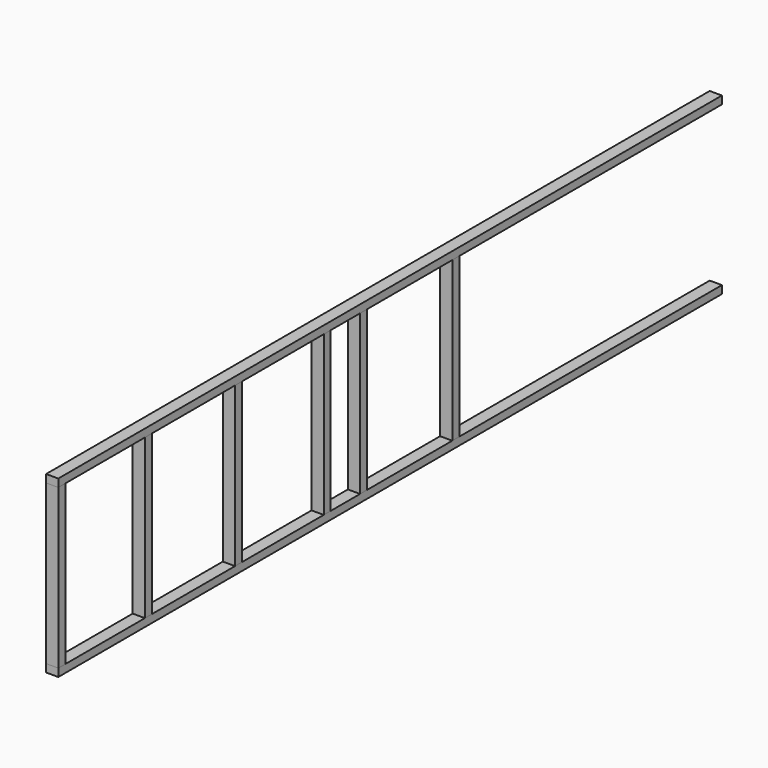
from build123d import *

# Parameters (mm, degrees)
F2_W     = 70
F2_H     = 45
F3_DEPTH = 2375
F4_W     = 50
F4_H     = 910.78125
F5_DEPTH = 70


with BuildPart() as f3:
    # F2 (on Front) → F3 (new body, symmetric)
    with BuildSketch(Plane.XZ):
        with Locations((-1245, 22.5)):
            Rectangle(F2_W, F2_H)
    extrude(amount=F3_DEPTH, both=True)


with BuildPart() as f3b:
    # F2 (on Front) → F3, piece 2 (new body, symmetric)
    with BuildSketch(Plane.XZ):
        with Locations((-1245, 978.28125)):
            Rectangle(F2_W, F2_H)
    extrude(amount=F3_DEPTH, both=True)


with BuildPart() as f5:
    # F4 (on face) → F5 (new body, through all)
    with BuildSketch(Plane(origin=(-1280, 0, 0), x_dir=(0, -1, 0), z_dir=(-1, 0, 0))):
        with Locations((2350, 500.390625)):
            Rectangle(F4_W, F4_H)
    extrude(amount=-F5_DEPTH)


with BuildPart() as f5b:
    # F4 (on face) → F5, piece 2 (new body, through all)
    with BuildSketch(Plane(origin=(-1280, 0, 0), x_dir=(0, -1, 0), z_dir=(-1, 0, 0))):
        with Locations((1730, 500.390625)):
            Rectangle(F4_W, F4_H)
    extrude(amount=-F5_DEPTH)


with BuildPart() as f5c:
    # F4 (on face) → F5, piece 3 (new body, through all)
    with BuildSketch(Plane(origin=(-1280, 0, 0), x_dir=(0, -1, 0), z_dir=(-1, 0, 0))):
        with Locations((1085, 500.390625)):
            Rectangle(F4_W, F4_H)
    extrude(amount=-F5_DEPTH)


with BuildPart() as f5d:
    # F4 (on face) → F5, piece 4 (new body, through all)
    with BuildSketch(Plane(origin=(-1280, 0, 0), x_dir=(0, -1, 0), z_dir=(-1, 0, 0))):
        with Locations((450, 500.390625)):
            Rectangle(F4_W, F4_H)
    extrude(amount=-F5_DEPTH)


with BuildPart() as f5e:
    # F4 (on face) → F5, piece 5 (new body, through all)
    with BuildSketch(Plane(origin=(-1280, 0, 0), x_dir=(0, -1, 0), z_dir=(-1, 0, 0))):
        with Locations((190, 500.390625)):
            Rectangle(F4_W, F4_H)
    extrude(amount=-F5_DEPTH)


with BuildPart() as f5f:
    # F4 (on face) → F5, piece 6 (new body, through all)
    with BuildSketch(Plane(origin=(-1280, 0, 0), x_dir=(0, -1, 0), z_dir=(-1, 0, 0))):
        with Locations((-470, 500.390625)):
            Rectangle(F4_W, F4_H)
    extrude(amount=-F5_DEPTH)


solid = Compound([f3.part, f3b.part, f5.part, f5b.part, f5c.part, f5d.part, f5e.part, f5f.part])
